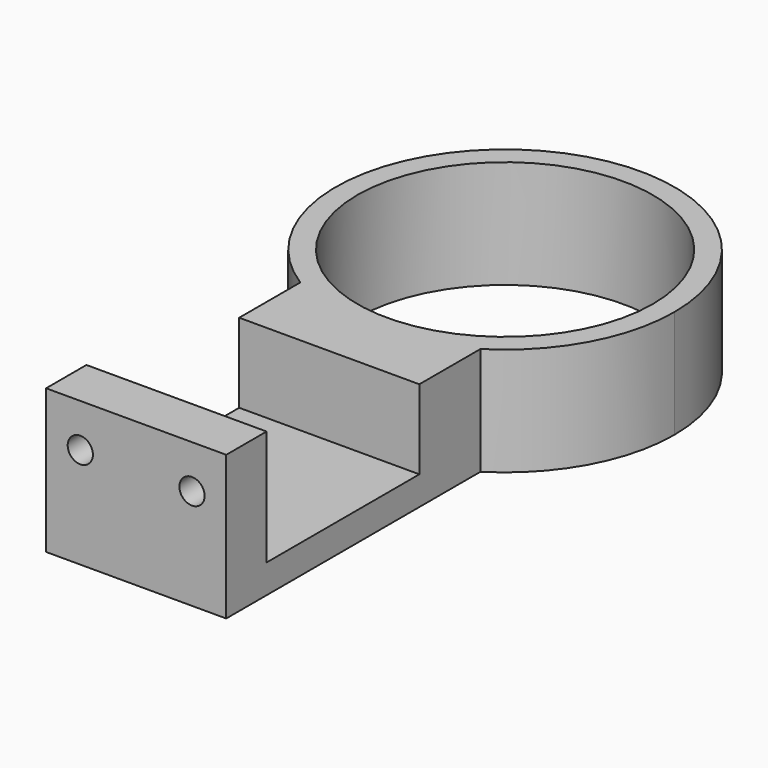
from build123d import *

# Parameters (mm, degrees)
F0_R     = 20.5
F1_DEPTH = 15
F0_W     = 25
F0_H     = 26.5
F2_DEPTH = 4
F0_H_2   = 7
F3_DEPTH = 20
F4_R     = 1.75
F5_DEPTH = 7


# Not quite as in the source:
# - a feature names something its author has since deleted; it is built from what else it names


with BuildPart() as f1:
    # F0 (on Top) → F1 (new body)
    with BuildSketch(Plane.XY):
        with BuildLine():
            ThreePointArc((12.5, -19.8997487421), (0, -23.5), (-12.5, -19.8997487421))
            Line((-12.5, -19.8997487421), (-12.5, -30.5))
            Line((-12.5, -30.5), (12.5, -30.5))
            Line((12.5, -30.5), (12.5, -19.8997487421))
        make_face()
        with BuildLine():
            ThreePointArc((23.5, 0), (-11.3688170009, 20.5669638012), (-12.5, -19.8997487421))
            ThreePointArc((-12.5, -19.8997487421), (0, -23.5), (12.5, -19.8997487421))
            ThreePointArc((12.5, -19.8997487421), (20.5669638012, -11.3688170009), (23.5, 0))
        make_face()
        Circle(F0_R, mode=Mode.SUBTRACT)
    extrude(amount=F1_DEPTH)

    # F0 (on Top) → F2 (join)
    with BuildSketch(Plane.XY):
        with BuildLine():
            ThreePointArc((12.5, -19.8997487421), (0, -23.5), (-12.5, -19.8997487421))
            Line((-12.5, -19.8997487421), (-12.5, -30.5))
            Line((-12.5, -30.5), (12.5, -30.5))
            Line((12.5, -30.5), (12.5, -19.8997487421))
        make_face()
        with Locations((0, -43.75)):
            Rectangle(F0_W, F0_H)
    extrude(amount=F2_DEPTH)

    # F0 (on Top) → F3 (join)
    with BuildSketch(Plane.XY):
        with Locations((0, -60.5)):
            Rectangle(F0_W, F0_H_2)
    extrude(amount=F3_DEPTH)

    # F4 (on face) → F5 (cut, through all)
    with BuildSketch(Plane.XZ.offset(64)):
        with Locations((-7.75, 14)):
            Circle(F4_R)
        with Locations((7.75, 14)):
            Circle(F4_R)
    extrude(amount=-F5_DEPTH, mode=Mode.SUBTRACT)


solid = f1.part
